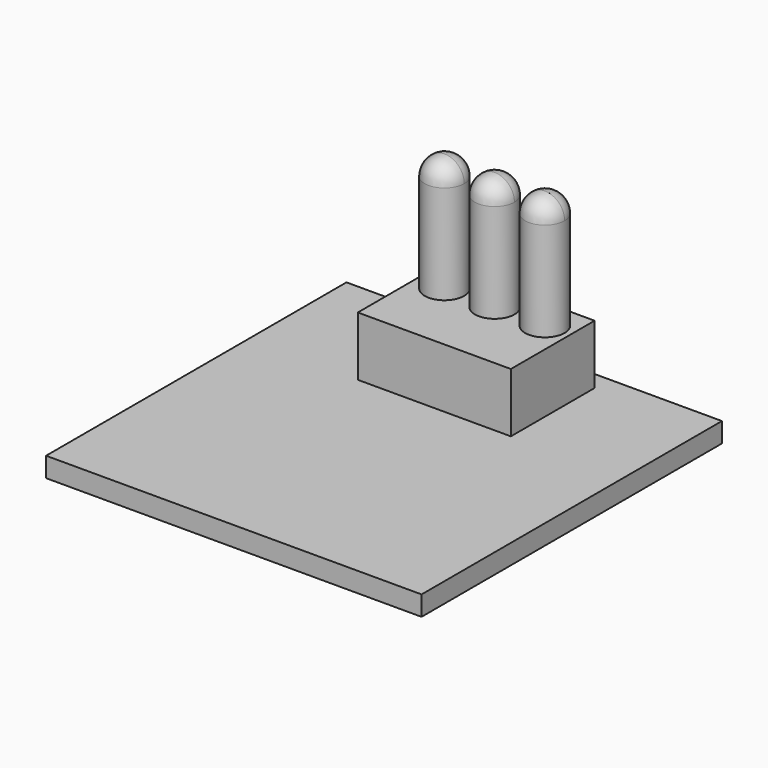
from build123d import *
from build123d import SkipClean  # not in build123d's __all__

# Parameters (mm, degrees)
F0_W     = 19
F0_H     = 19
F1_DEPTH = 1
F2_W     = 7.7446724754
F2_H     = 5.2963567432
F3_DEPTH = 3
F4_R     = 1
F5_DEPTH = 5


with BuildPart() as f1:
    # F0 (on Top) → F1 (new body)
    with BuildSketch(Plane.XY):
        with Locations((0, -7)):
            Rectangle(F0_W, F0_H)
    extrude(amount=F1_DEPTH)


with BuildPart() as f3:
    # F2 (on face) → F3 (new body)
    with BuildSketch(Plane.XY.offset(1)):
        with Locations((-0.065915403, -1.0850959225)):
            Rectangle(F2_W, F2_H)
    extrude(amount=F3_DEPTH)


with BuildPart() as f5:
    # F4 (on face) → F5 (new body)
    with BuildSketch(Plane.XY.offset(4)):
        with Locations((-2.54, 0)):
            Circle(F4_R)
    extrude(amount=F5_DEPTH)

    # F6 (on Front) → F7, piece 3 (revolve)
    with BuildSketch(Plane.XZ):
        with BuildLine():
            Line((-3.54, 9), (-1.54, 9))
            ThreePointArc((-1.54, 9), (-2.54, 10), (-3.54, 9))
        make_face()
    with SkipClean():  # cleaning this boolean's faces spoils the solid; the shape is the same uncleaned
        revolve(axis=Axis((0, 0, 9), (1, 0, 0)))


with BuildPart() as f5b:
    # F4 (on face) → F5, piece 2 (new body)
    with BuildSketch(Plane.XY.offset(4)):
        Circle(F4_R)
    extrude(amount=F5_DEPTH)

    # F6 (on Front) → F7 (revolve)
    with BuildSketch(Plane.XZ):
        with BuildLine():
            Line((-1, 9), (1, 9))
            ThreePointArc((1, 9), (0, 10), (-1, 9))
        make_face()
    with SkipClean():  # cleaning this boolean's faces spoils the solid; the shape is the same uncleaned
        revolve(axis=Axis((0, 0, 9), (1, 0, 0)))


with BuildPart() as f5c:
    # F4 (on face) → F5, piece 3 (new body)
    with BuildSketch(Plane.XY.offset(4)):
        with Locations((2.54, 0)):
            Circle(F4_R)
    extrude(amount=F5_DEPTH)

    # F6 (on Front) → F7, piece 2 (revolve)
    with BuildSketch(Plane.XZ):
        with BuildLine():
            Line((1.54, 9), (3.54, 9))
            ThreePointArc((3.54, 9), (2.54, 10), (1.54, 9))
        make_face()
    with SkipClean():  # cleaning this boolean's faces spoils the solid; the shape is the same uncleaned
        revolve(axis=Axis((0, 0, 9), (1, 0, 0)))


solid = Compound([f1.part, f3.part, f5.part, f5b.part, f5c.part])
